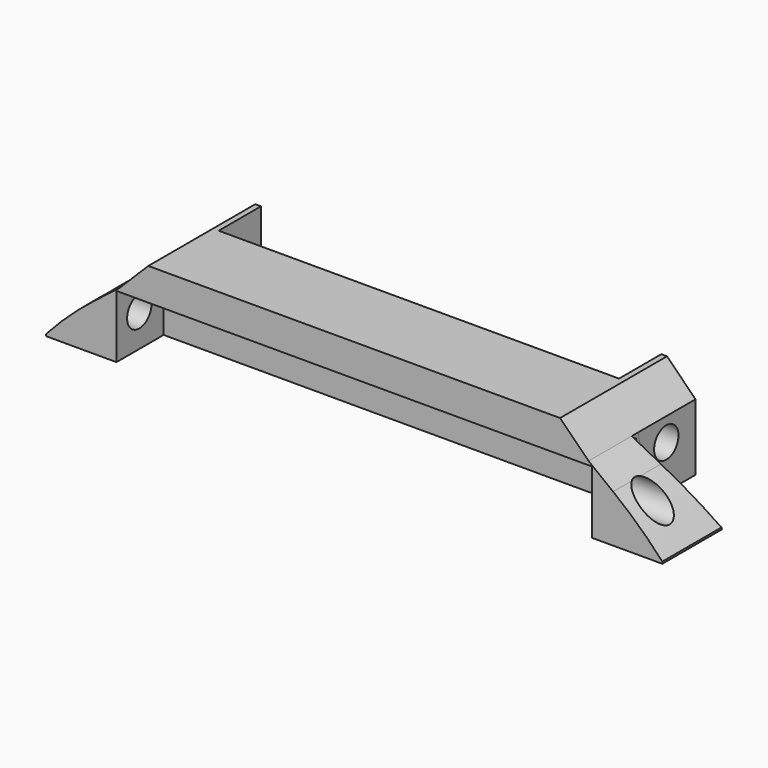
from build123d import *

# Parameters (mm, degrees)
F1_R           = 1.6
F2_DEPTH       = 33
F2_DEPTH_BACK  = 33
F4_DEPTH       = 62.0586978075
F8_W           = 6.3
F8_H           = 7
F9_DEPTH       = 25
F9_DEPTH_BACK  = 25
F10_R          = 1.6
F11_DEPTH      = 32.4035001
F11_DEPTH_BACK = 32.4035001
F13_DEPTH      = 3
F14_W          = 42.103
F14_H          = 3
F15_DEPTH      = 2
F16_SIZE       = 2.99999
F18_DEPTH      = 25


# Not quite as in the source:
# - a fillet or chamfer is up to 0.001 mm smaller than in the source, because OpenCascade refuses the exact size
# - a pattern or mirror of a feature is missing from the dataset's text; its kind, count and spacing are read off the source's solid


with BuildPart() as f2:
    # F1 (on offset) → F2 (new body, two sides)
    with BuildSketch(Plane.YZ.offset(-40)) as f2_sk:
        with BuildLine():
            Line((-55.5576978075, 47), (-62.0576978075, 47))
            Line((-62.0576978075, 47), (-62.0576978075, 40))
            Line((-62.0576978075, 40), (-53.0576978075, 40))
            ThreePointArc((-53.0576978075, 40), (-53.9183376958, 41.7448320543), (-54.7576978075, 43.5))
            ThreePointArc((-54.7576978075, 43.5), (-55.1675152463, 45.247756014), (-55.5576978075, 47))
        make_face()
        with Locations((-59.0576978075, 43.5)):
            Circle(F1_R, mode=Mode.SUBTRACT)
    extrude(amount=F2_DEPTH)
    extrude(f2_sk.sketch, amount=-F2_DEPTH_BACK)

    # F3 (on Front) → F4 (cut, through all)
    with BuildSketch(Plane.XZ):
        with BuildLine():
            ThreePointArc((-72.4025, 40.2057909187), (-69.9229908245, 42.7170557867), (-67.2317861301, 45))
            Line((-67.2317861301, 45), (-64.6515, 47))
            Line((-64.6515, 47), (-77.5247141719, 47))
            Line((-77.5247141719, 47), (-77.5247141719, 39.4350364804))
            Line((-77.5247141719, 39.4350364804), (-72.4025, 39.4350364804))
            Line((-72.4025, 39.4350364804), (-72.4025, 40.2057909187))
        make_face()
        with BuildLine():
            Line((-7.5975, 40.2057909187), (-7.5975, 39.4350364804))
            Line((-7.5975, 39.4350364804), (-2.4752858281, 39.4350364804))
            Line((-2.4752858281, 39.4350364804), (-2.4752858281, 47))
            Line((-2.4752858281, 47), (-15.3485, 47))
            Line((-15.3485, 47), (-12.7682138699, 45))
            ThreePointArc((-12.7682138699, 45), (-10.0770091755, 42.7170557867), (-7.5975, 40.2057909187))
        make_face()
    extrude(amount=F4_DEPTH, mode=Mode.SUBTRACT)

    # F6 (on offset) → F7 (join, up to the next surface of F2)
    with BuildSketch(Plane.XZ.offset(48)):
        Polygon((-64.6515, 47), (-64.6515, 44.9052631579), (-64.6515, 40), (-61.0515, 40), (-61.0515, 44.9052631579), (-61.0515, 47), align=None)
    f7 = extrude(until=Until.NEXT)

    # F7_copies: F7 across plane
    add(f7.mirror(Plane(origin=(-40.000004, 0, 3e-06), x_dir=(0, 0, 1), z_dir=(1, 0, 0))))

    # F8 (on offset) → F9 (cut, two sides)
    with BuildSketch(Plane.YZ.offset(-40)) as f9_sk:
        with Locations((-59.0076978075, 43.1)):
            Rectangle(F8_W, F8_H)
    extrude(amount=-F9_DEPTH, mode=Mode.SUBTRACT)
    extrude(f9_sk.sketch, amount=F9_DEPTH_BACK, mode=Mode.SUBTRACT)

    # F10 (on offset) → F11 (cut, two sides)
    with BuildSketch(Plane.YZ.offset(-40)) as f11_sk:
        with Locations((-51.845, 44.56195746)):
            Circle(F10_R)
    extrude(amount=-F11_DEPTH, mode=Mode.SUBTRACT)
    extrude(f11_sk.sketch, amount=F11_DEPTH_BACK, mode=Mode.SUBTRACT)

    # F12 (on face) → F13 (join)
    with BuildSketch(Plane.XY.offset(47)):
        Polygon((-64.6515, -48.0000000008), (-64.6515, -55.5576978083), (-64.6515, -62.0576978075), (-15.3485, -62.0576978075), (-15.3485, -55.5576978075), (-15.3485, -48.0000000007), (-18.9485, -48), (-18.9485, -55.5576978084), (-61.0515, -55.5576978075), (-61.0515, -48.0000000007), align=None)
    extrude(amount=F13_DEPTH)

    # F14 (on face) → F15 (join)
    with BuildSketch(Plane(origin=(0, -55.5576978075, 0), x_dir=(-1, 0, 0), z_dir=(0, 1, 0))):
        with Locations((40, 48.5)):
            Rectangle(F14_W, F14_H)
    extrude(amount=F15_DEPTH)

    # F16 (size 3 in the source; OpenCascade refuses exactly that, so slightly less here)
    f16_edges = [f2.edges().sort_by_distance(p)[0] for p in [
        (-64.6515, -55.028849, 50),
        (-15.3485, -55.028849, 50),
    ]]
    chamfer(f16_edges, length=F16_SIZE)

    # F17 (on face) → F18 (cut)
    with BuildSketch(Plane(origin=(-64.6515, 0, 0), x_dir=(0, -1, 0), z_dir=(-1, 0, 0))):
        Polygon((56.3939474523, 47), (55.5576978075, 47), (53.0576978076, 40), (54.2201250792, 40), align=None)
    f18 = extrude(amount=F18_DEPTH, mode=Mode.SUBTRACT)

    # F18_copies: F18 across plane
    add(f18.mirror(Plane(origin=(-40, 0, 0), x_dir=(0, 0, 1), z_dir=(1, 0, 0))), mode=Mode.SUBTRACT)


solid = f2.part
